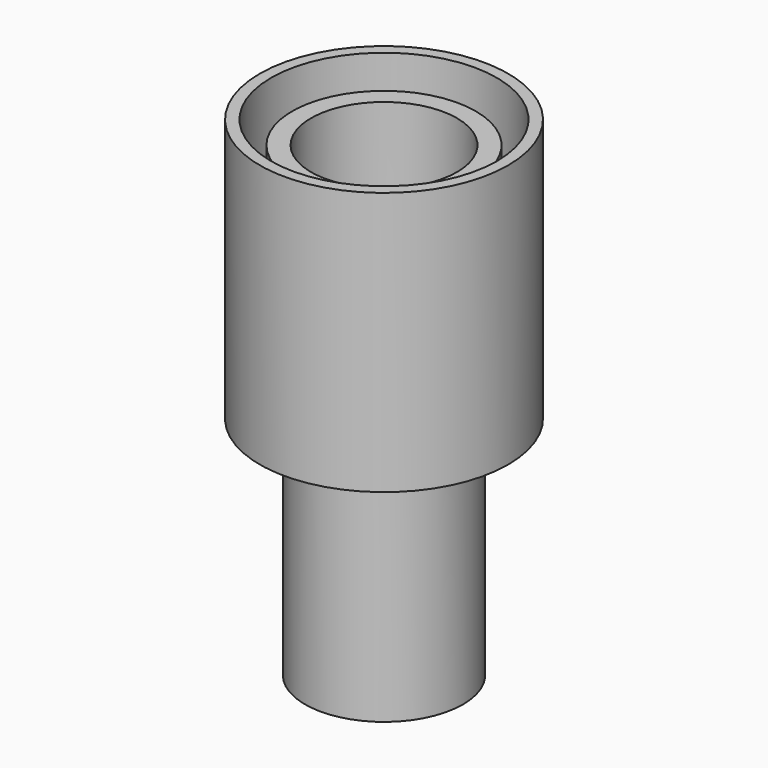
from build123d import *

# Parameters (mm, degrees)
F0_R      = 16.5
F1_DEPTH  = 5
F2_R      = 16.5
F2_R_2    = 15
F3_DEPTH  = 30
F4_R      = 12.2
F4_R_2    = 9.7
F5_DEPTH  = 27
F6_R      = 10.5
F7_DEPTH  = 30
F8_R      = 9.5
F8_R_2    = 8
F8_R_3    = 6.5
F9_DEPTH  = 30
F10_DEPTH = 30
F11_SIZE2 = 0.610917
F11_SIZE  = 34.99999


# Not quite as in the source:
# - a fillet or chamfer is up to 0.001 mm smaller than in the source, because OpenCascade refuses the exact size


with BuildPart() as f1:
    # F0 (on Top) → F1 (new body)
    with BuildSketch(Plane.XY):
        Circle(F0_R)
    extrude(amount=F1_DEPTH)

    # F2 (on face) → F3 (join)
    with BuildSketch(Plane.XY.offset(5)):
        Circle(F2_R)
        Circle(F2_R_2, mode=Mode.SUBTRACT)
    extrude(amount=F3_DEPTH)

    # F4 (on face) → F5 (join)
    with BuildSketch(Plane.XY.offset(5)):
        Circle(F4_R)
        Circle(F4_R_2, mode=Mode.SUBTRACT)
    extrude(amount=F5_DEPTH)

    # F6 (on face) → F7 (join)
    with BuildSketch(Plane(origin=(0, 0, 0), x_dir=(1, 0, 0), z_dir=(0, 0, -1))):
        Circle(F6_R)
    extrude(amount=F7_DEPTH)

    # F8 (on face) → F9 (cut)
    with BuildSketch(Plane(origin=(0, 0, -30), x_dir=(1, 0, 0), z_dir=(0, 0, -1))):
        Circle(F8_R)
        Circle(F8_R_2, mode=Mode.SUBTRACT)
        Circle(F8_R_3)
    extrude(amount=-F9_DEPTH, mode=Mode.SUBTRACT)

    # F10 (cut): a face of the model
    f10_faces = [f1.faces().sort_by_distance(p)[0] for p in [
        (0, 0, 0),
    ]]
    extrude(f10_faces, amount=-F10_DEPTH, mode=Mode.SUBTRACT)

    # F11 (size 35 and 0.6109272725 in the source; OpenCascade refuses exactly that, so slightly less here)
    f11_edges = [f1.edges().sort_by_distance(p)[0] for p in [
        (-6.5, 0, 5),
    ]]
    f11_side = f1.faces().sort_by_distance((-6.5, 0, -12.5))[0]
    chamfer(f11_edges, length=F11_SIZE, length2=F11_SIZE2, reference=f11_side)


solid = f1.part
